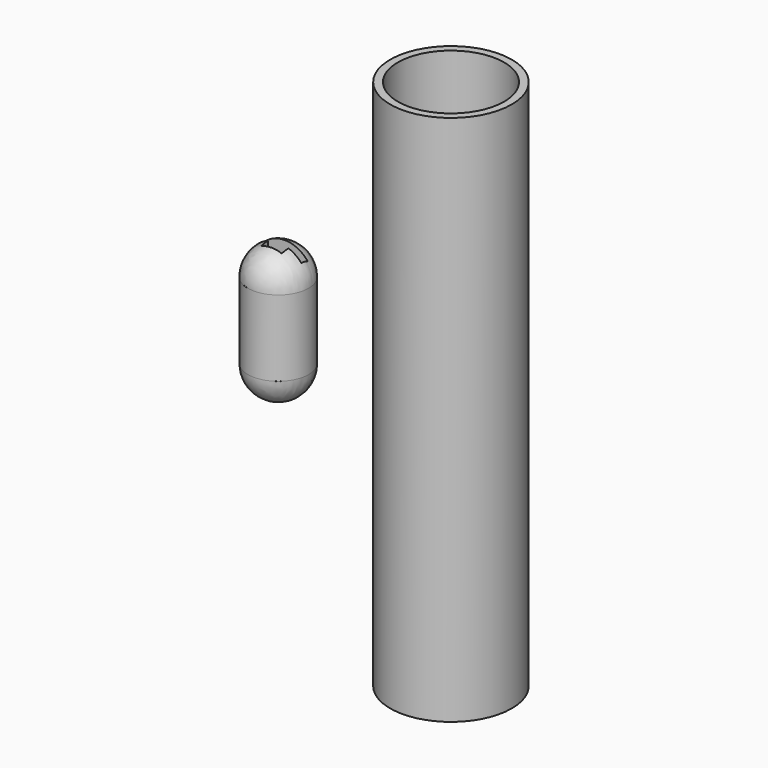
from build123d import *

# Parameters (mm, degrees)
F5_ANGLE       = 180
F6_DEPTH       = 18
F7_REACH       = 9.8039879523
F8_ANGLE       = 180
F9_REACH       = 9.8039879523
F0_R           = 5.08
F10_DEPTH      = 6.35
F10_DEPTH_BACK = 6.35
F11_R          = 10.16
F11_R_2        = 8.89
F12_DEPTH      = 44.45


# Not quite as in the source:
# - after a boolean that leaves OpenCascade's solid faulty, fix() repairs it
# - an extrude ends at something that could not be found from the text; its depth is read off the source's solid
# - ends of sketch curves that miss each other by under 0.0002 mm in the source are joined


with BuildPart() as f5:
    # F3 (on offset) → F5 (revolve)
    with BuildSketch(Plane.XY.offset(6.35)):
        with BuildLine():
            Line((9.3459e-06, 1.341628), (0, 5.08))
            ThreePointArc((0, 5.08), (-5.08, -1.27e-05), (2.54e-05, -5.08))
            Line((2.54e-05, -5.08), (1.61626e-05, -1.3850366))
            Line((1.61626e-05, -1.3850366), (-1.7108932, -1.3850366))
            Line((-1.7108932, -1.3850366), (-1.7108932, 0))
            Line((-1.7108932, 0), (-3.8563804, 0))
            Line((-3.8563804, 0), (-3.8563804, 1.341628))
            Line((-3.8563804, 1.341628), (9.3459e-06, 1.341628))
        make_face()
        Polygon((0, 0), (0, 1.341628), (-3.8563804, 1.341628), (-3.8563804, 0), (-1.7108932, 0), (-1.7108932, -1.3850366), (1.61626e-05, -1.3850366), align=None)
    revolve(axis=Axis((1.27e-05, 0, 6.35), (-2.5e-06, 1, 0)), revolution_arc=F5_ANGLE)

    # F3 (on offset) → F6 (cut, through all)
    with BuildSketch(Plane.XY.offset(6.35)):
        Polygon((3.8563804, 1.341628), (0, 1.341628), (0, 0), (1.61626e-05, -1.3850366), (1.710944, -1.3850366), (1.710944, 0), (3.8563804, 0), align=None)
        Polygon((0, 0), (0, 1.341628), (-3.8563804, 1.341628), (-3.8563804, 0), (-1.7108932, 0), (-1.7108932, -1.3850366), (1.61626e-05, -1.3850366), align=None)
    extrude(amount=-F6_DEPTH, mode=Mode.SUBTRACT)

    add(f5.part.fix(), mode=Mode.REPLACE)

    f7_end = f5.faces().sort_by_distance((1.27e-05, 0, 11.4300127))[0]
    # F3 (on offset) → F7 (cut, up to a face of the model that its end follows)
    with BuildSketch(Plane.XY.offset(6.35)):
        Polygon((0, 0), (0, 1.341628), (-3.8563804, 1.341628), (-3.8563804, 0), (-1.7108932, 0), (-1.7108932, -1.3850366), (1.61626e-05, -1.3850366), align=None)
        Polygon((3.8563804, 1.341628), (0, 1.341628), (0, 0), (1.61626e-05, -1.3850366), (1.710944, -1.3850366), (1.710944, 0), (3.8563804, 0), align=None)
    f7_long = extrude(amount=F7_REACH, mode=Mode.PRIVATE)
    add(split(f7_long, bisect_by=f7_end, keep=Keep.BOTTOM, mode=Mode.PRIVATE), mode=Mode.SUBTRACT)


with BuildPart() as f8:
    # F4 (on offset) → F8 (revolve)
    with BuildSketch(Plane.XY.offset(-6.35)):
        with BuildLine():
            Line((9.3459e-06, 1.341628), (0, 5.08))
            ThreePointArc((0, 5.08), (-5.08, -1.27e-05), (2.54e-05, -5.08))
            Line((2.54e-05, -5.08), (1.61626e-05, -1.3850366))
            Line((1.61626e-05, -1.3850366), (-1.7108932, -1.3850366))
            Line((-1.7108932, -1.3850366), (-1.7108932, 0))
            Line((-1.7108932, 0), (-3.8563804, 0))
            Line((-3.8563804, 0), (-3.8563804, 1.341628))
            Line((-3.8563804, 1.341628), (9.3459e-06, 1.341628))
        make_face()
        Polygon((0, 0), (0, 1.341628), (-3.8563804, 1.341628), (-3.8563804, 0), (-1.7108932, 0), (-1.7108932, -1.3850366), (1.61626e-05, -1.3850366), align=None)
    revolve(axis=Axis((1.27e-05, 0, -6.35), (2.5e-06, -1, 0)), revolution_arc=F8_ANGLE)

    f9_end = f8.faces().sort_by_distance((1.27e-05, 0, -11.4300127))[0]
    # F4 (on offset) → F9 (cut, up to a face of the model that its end follows)
    with BuildSketch(Plane.XY.offset(-6.35)):
        Polygon((3.8563804, 1.341628), (0, 1.341628), (0, 0), (1.61626e-05, -1.3850366), (1.710944, -1.3850366), (1.710944, 0), (3.8563804, 0), align=None)
        Polygon((0, 0), (0, 1.341628), (-3.8563804, 1.341628), (-3.8563804, 0), (-1.7108932, 0), (-1.7108932, -1.3850366), (1.61626e-05, -1.3850366), align=None)
    f9_long = extrude(amount=-F9_REACH, mode=Mode.PRIVATE)
    add(split(f9_long, bisect_by=f9_end, keep=Keep.BOTTOM, mode=Mode.PRIVATE), mode=Mode.SUBTRACT)


with BuildPart() as f10:
    # F0 (on Top) → F10 (new body, two sides)
    with BuildSketch(Plane.XY) as f10_sk:
        Circle(F0_R)
        Polygon((-3.856369298, 1.3546424612), (0, 1.3546424612), (3.856369298, 1.3546424612), (3.856369298, 0.013024848), (1.7109218004, 0.013024848), (1.7109218004, -1.3720089252), (0, -1.3720089252), (-1.7109218004, -1.3720089252), (-1.7109218004, 0.013024848), (-3.856369298, 0.013024848), align=None, mode=Mode.SUBTRACT)
    extrude(amount=F10_DEPTH)
    extrude(f10_sk.sketch, amount=-F10_DEPTH_BACK)


with BuildPart() as f12:
    # F11 (on Top) → F12 (new body, symmetric)
    with BuildSketch(Plane.XY):
        with Locations((28.880469501, 0)):
            Circle(F11_R)
        with Locations((28.880469501, 0)):
            Circle(F11_R_2, mode=Mode.SUBTRACT)
    extrude(amount=F12_DEPTH, both=True)


solid = Compound([f5.part, f8.part, f10.part, f12.part])
